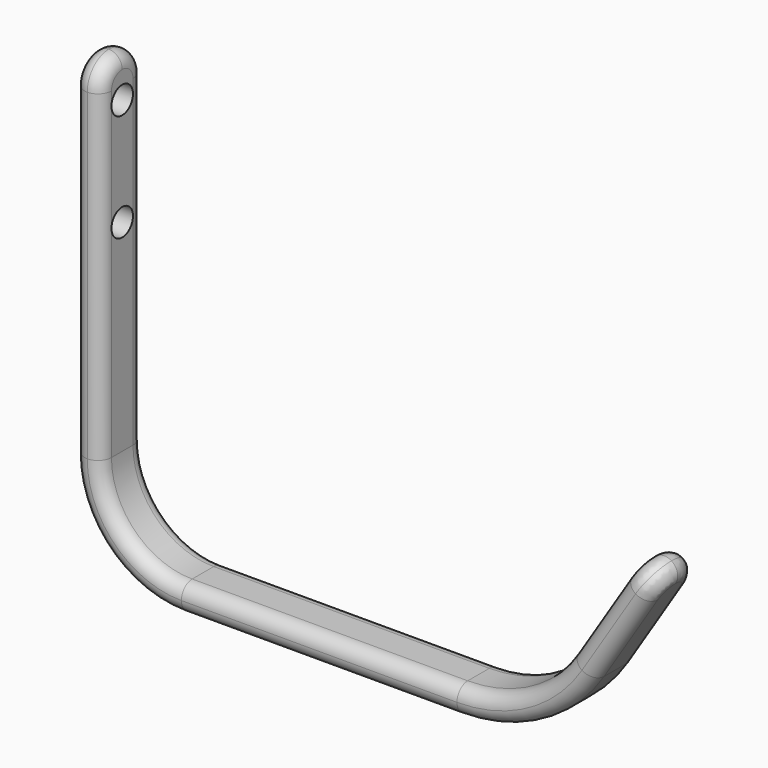
from build123d import *

# Parameters (mm, degrees)
F1_DEPTH    = 6.35
F2_T1_DEPTH = 38.1
F3_T1_DEPTH = 38.1
F5_R        = 3.17499
F6_R        = 3.175
F7_DEPTH    = 25.4


# Not quite as in the source:
# - a fillet or chamfer that OpenCascade refuses, or shapes differently, is made with other operations: its cross-section is extruded or revolved along the edge and cut away or added
# - a fillet or chamfer is up to 0.001 mm smaller than in the source, because OpenCascade refuses the exact size
# - a feature of the source that left no trace in its solid (it failed there, or was rolled back) is left out


with BuildPart() as f1:
    # F0 (on Front) → F1 (new body, symmetric)
    with BuildSketch(Plane.XZ):
        with BuildLine():
            Line((-81.1784485418, -7.2266137339), (-81.1784485418, 75.3233862661))
            Line((-81.1784485418, 75.3233862661), (-87.5284485418, 75.3233862661))
            Line((-87.5284485418, 75.3233862661), (-87.5284485418, -7.2266137339))
            ThreePointArc((-87.5284485418, -7.2266137339), (-80.0889607839, -25.1871259761), (-62.1284485418, -32.6266137339))
            Line((-62.1284485418, -32.6266137339), (2.9360103709, -32.6266137339))
            ThreePointArc((2.9360103709, -32.6266137339), (21.3157063883, -27.9002077014), (35.1353023462, -14.8936360074))
            Line((35.1353023462, -14.8936360074), (51.1881001208, 10.4850725552))
            Line((51.1881001208, 10.4850725552), (45.8215514582, 13.8795762674))
            Line((45.8215514582, 13.8795762674), (29.7687536837, -11.4991322951))
            ThreePointArc((29.7687536837, -11.4991322951), (18.2524237187, -22.3379420402), (2.9360103709, -26.2766137339))
            Line((2.9360103709, -26.2766137339), (-62.1284485418, -26.2766137339))
            ThreePointArc((-62.1284485418, -26.2766137339), (-75.5988327234, -20.6969979155), (-81.1784485418, -7.2266137339))
        make_face()
    extrude(amount=F1_DEPTH, both=True)

    # F2: fillet of radius 6.35 on 2 edges, made by hand

    # F2_s2 → F2_t1 (cut)
    with BuildSketch(Plane.YZ.offset(-103.4034485418)):
        with BuildLine():
            ThreePointArc((0, 75.3233862661), (4.4901280605, 73.4635143266), (6.35, 68.9733862661))
            Line((6.35, 68.9733862661), (6.35, 75.3233862661))
            Line((6.35, 75.3233862661), (0, 75.3233862661))
        make_face()
        with BuildLine():
            ThreePointArc((0, 75.3233862661), (-4.4901280605, 73.4635143266), (-6.35, 68.9733862661))
            Line((-6.35, 68.9733862661), (-6.35, 75.3233862661))
            Line((-6.35, 75.3233862661), (0, 75.3233862661))
        make_face()
    extrude(amount=F2_T1_DEPTH, mode=Mode.SUBTRACT)

    # F3: fillet of radius 6.35 on 2 edges, made by hand

    # F3_s2 → F3_t1 (cut)
    with BuildSketch(Plane(origin=(45.2399237114, 0, -28.6156147341), x_dir=(0, 1, 0), z_dir=(-0.8451257736, 0, 0.5345675137))):
        with BuildLine():
            ThreePointArc((-6.35, -29.8747004693), (-4.4901280605, -34.3648285299), (0, -36.2247004693))
            Line((0, -36.2247004693), (-6.35, -36.2247004693))
            Line((-6.35, -36.2247004693), (-6.35, -29.8747004693))
        make_face()
        with BuildLine():
            ThreePointArc((6.35, -29.8747004693), (4.4901280605, -34.3648285299), (0, -36.2247004693))
            Line((0, -36.2247004693), (6.35, -36.2247004693))
            Line((6.35, -36.2247004693), (6.35, -29.8747004693))
        make_face()
    extrude(amount=F3_T1_DEPTH, mode=Mode.SUBTRACT)

    # F5 (radius 3.175 in the source; OpenCascade refuses exactly that, so slightly less here)
    f5_edges = [f1.edges().sort_by_distance(p)[0] for p in [
        (-81.178449, -6.35, 30.873386),
        (18.252424, 6.35, -22.337942),
        (18.252424, -6.35, -22.337942),
        (41.464449, 6.35, -4.887556),
        (21.315706, 6.35, -27.900208),
        (-29.596219, 6.35, -32.626614),
        (-80.088961, 6.35, -25.187126),
        (-87.528449, 6.35, 30.873386),
        (-81.178449, 6.35, 30.873386),
        (-75.598833, 6.35, -20.696998),
        (-29.596219, 6.35, -26.276614),
        (36.097901, 6.35, -1.493052),
        (-29.596219, -6.35, -26.276614),
        (41.464449, -6.35, -4.887556),
        (21.315706, -6.35, -27.900208),
        (-29.596219, -6.35, -32.626614),
        (-80.088961, -6.35, -25.187126),
        (-87.528449, -6.35, 30.873386),
        (-75.598833, -6.35, -20.696998),
        (36.097901, -6.35, -1.493052),
        (44.827324, 4.490128, 12.307751),
        (44.827324, -4.490128, 12.307751),
        (50.193873, 4.490128, 8.913247),
        (50.193873, -4.490128, 8.913247),
        (-87.528449, -4.490128, 73.463514),
        (-87.528449, 4.490128, 73.463514),
        (-81.178449, 4.490128, 73.463514),
        (-81.178449, -4.490128, 73.463514),
    ]]
    fillet(f5_edges, radius=F5_R)

    # F6 (on face) → F7 (cut)
    with BuildSketch(Plane(origin=(-87.5284485418, 0, 0), x_dir=(0, -1, 0), z_dir=(-1, 0, 0))):
        with Locations((0, 65.7983862661)):
            Circle(F6_R)
        with Locations((0, 40.3983862661)):
            Circle(F6_R)
    extrude(amount=-F7_DEPTH, mode=Mode.SUBTRACT)


solid = f1.part
